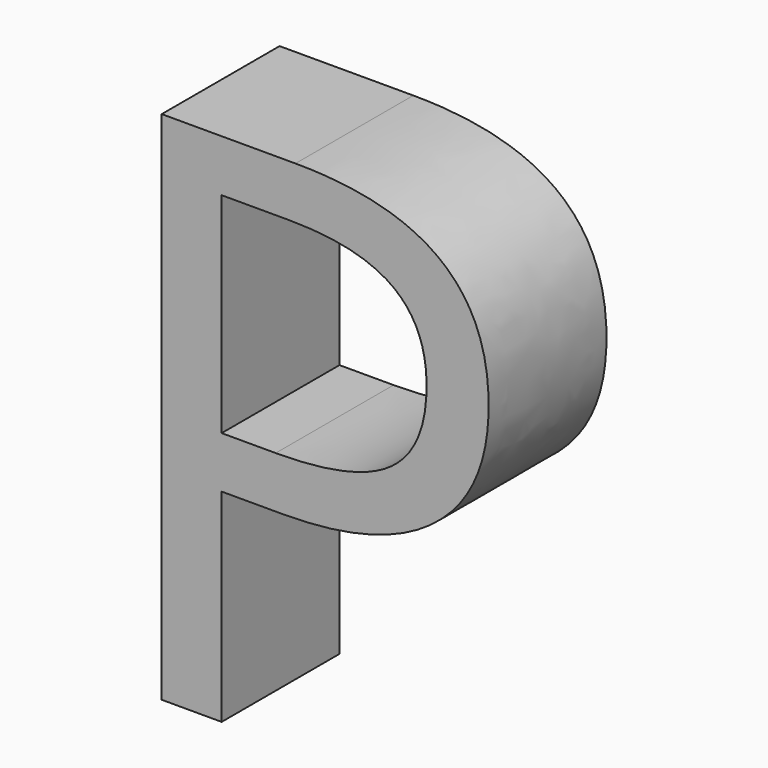
from build123d import *

# Parameters (mm, degrees)
F0_TEXT_SIZE = 49.0367050386
F1_DEPTH     = 10


# Not quite as in the source:
# - Text() gives the source's letters only with a copy of the font that has no kerning and outlines rounded to 1/6400 em; it was checked with that copy


with BuildPart() as f1:
    # F0 (on Front) → F1 (new body)
    with BuildSketch(Plane.XZ):
        with Locations((-30.1882215394, 0)):
            Text('P', F0_TEXT_SIZE, font='Open Sans', text_align=(TextAlign.LEFT, TextAlign.BOTTOM))
    extrude(amount=F1_DEPTH)


solid = f1.part
